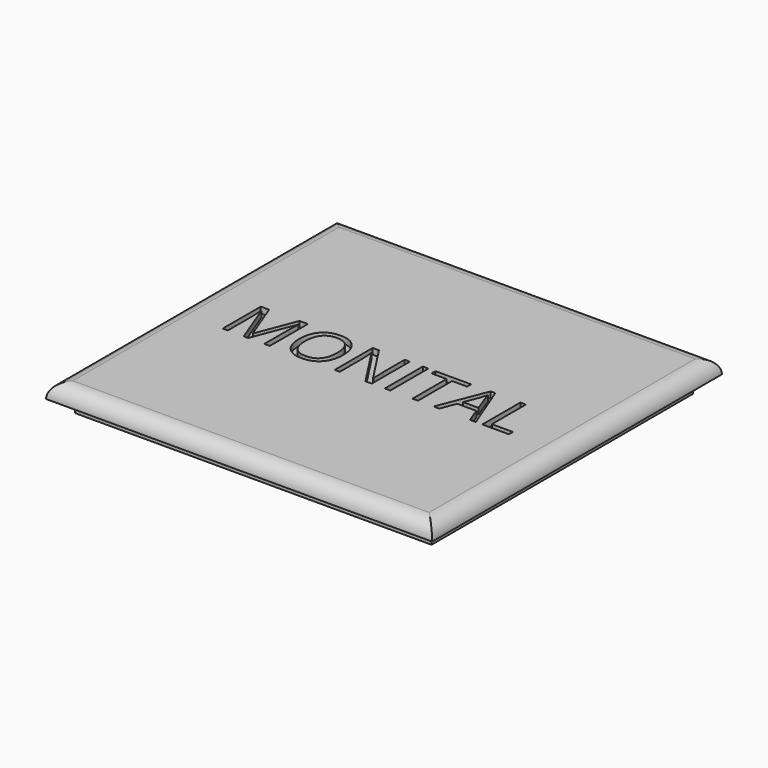
from build123d import *

# Parameters (mm, degrees)
F0_W         = 65
F0_H         = 61
F1_DEPTH     = 2.5
F2_R         = 2.49999
F3_TEXT_SIZE = 11.2076211824
F4_DEPTH     = 1
F5_W         = 60
F5_H         = 55
F6_DEPTH     = 2.5


# Not quite as in the source:
# - a fillet or chamfer is up to 0.001 mm smaller than in the source, because OpenCascade refuses the exact size
# - Text() gives the source's letters only with a copy of the font that has no kerning and outlines rounded to 1/6400 em; it was checked with that copy


with BuildPart() as f1:
    # F0 (on Top) → F1 (new body)
    with BuildSketch(Plane.XY):
        Rectangle(F0_W, F0_H)
    extrude(amount=F1_DEPTH)

    # F2 (radius 2.5 in the source; OpenCascade refuses exactly that, so slightly less here)
    f2_edges = [f1.edges().sort_by_distance(p)[0] for p in [
        (0, -30.5, 2.5),
        (-32.5, 0, 2.5),
        (0, 30.5, 2.5),
        (32.5, 0, 2.5),
    ]]
    fillet(f2_edges, radius=F2_R)

    # F3 (on face) → F4 (cut)
    with BuildSketch(Plane.XY.offset(2.5)):
        with Locations((-25, -4.0694872513)):
            Text('MONITAL', F3_TEXT_SIZE, font='Open Sans', text_align=(TextAlign.LEFT, TextAlign.BOTTOM))
    extrude(amount=-F4_DEPTH, mode=Mode.SUBTRACT)

    # F5 (on face) → F6 (join)
    with BuildSketch(Plane(origin=(0, 0, 0), x_dir=(1, 0, 0), z_dir=(0, 0, -1))):
        Rectangle(F5_W, F5_H)
    extrude(amount=F6_DEPTH)


solid = f1.part
